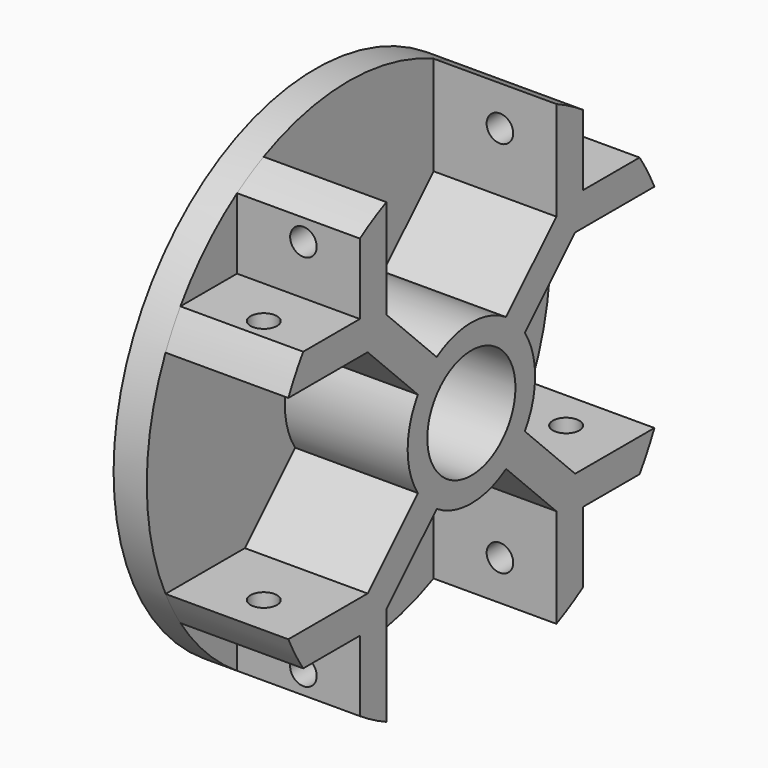
from build123d import *

# Parameters (mm, degrees)
F0_R            = 19
F1_DEPTH        = 2.5
F3_DEPTH        = 9.25
F4_R            = 1
F5_DEPTH        = 20
F5_COPIES_COUNT = 3
F5_COPIES_ANGLE = 180
F6_R            = 1
F7_DEPTH        = 20
F8_R            = 3
F9_DEPTH        = 2
F10_DEPTH       = 2
F11_R           = 4.15
F12_DEPTH       = 11.75


# Not quite as in the source:
# - a pattern or mirror of a feature is missing from the dataset's text; its kind, count and spacing are read off the source's solid


with BuildPart() as f1:
    # F0 (on Right) → F1 (new body)
    with BuildSketch(Plane.YZ):
        Circle(F0_R)
    extrude(amount=F1_DEPTH)

    # F2 (on face) → F3 (join)
    with BuildSketch(Plane.YZ.offset(2.5)):
        with BuildLine():
            ThreePointArc((-8, 17.2336879396), (-9.2763958902, 16.5815704711), (-10.5, 15.8350876221))
            Line((-10.5, 15.8350876221), (-10.5, 10.5))
            Line((-10.5, 10.5), (-15.8350876221, 10.5))
            ThreePointArc((-15.8350876221, 10.5), (-16.5815704711, 9.2763958902), (-17.2336879396, 8))
            Line((-17.2336879396, 8), (-9.767766953, 8))
            Line((-9.767766953, 8), (-5.0334316447, 3.2656646917))
            ThreePointArc((-5.0334316447, 3.2656646917), (-4.2426406871, 4.2426406871), (-3.2656646917, 5.0334316447))
            Line((-3.2656646917, 5.0334316447), (-8, 9.767766953))
            Line((-8, 9.767766953), (-8, 17.2336879396))
        make_face()
        with BuildLine():
            ThreePointArc((3.2656646917, 5.0334316447), (0, 6), (-3.2656646917, 5.0334316447))
            ThreePointArc((-3.2656646917, 5.0334316447), (-4.2426406871, 4.2426406871), (-5.0334316447, 3.2656646917))
            ThreePointArc((-5.0334316447, 3.2656646917), (-6, 0), (-5.0334316447, -3.2656646917))
            ThreePointArc((-5.0334316447, -3.2656646917), (-4.2426406871, -4.2426406871), (-3.2656646917, -5.0334316447))
            ThreePointArc((-3.2656646917, -5.0334316447), (0, -6), (3.2656646917, -5.0334316447))
            ThreePointArc((3.2656646917, -5.0334316447), (4.2426406871, -4.2426406871), (5.0334316447, -3.2656646917))
            ThreePointArc((5.0334316447, -3.2656646917), (5.7532855773, -1.7028520388), (6, 0))
            ThreePointArc((6, 0), (5.7532855773, 1.7028520388), (5.0334316447, 3.2656646917))
            ThreePointArc((5.0334316447, 3.2656646917), (4.2426406871, 4.2426406871), (3.2656646917, 5.0334316447))
        make_face()
        with BuildLine():
            ThreePointArc((10.5, 15.8350876221), (9.2763958902, 16.5815704711), (8, 17.2336879396))
            Line((8, 17.2336879396), (8, 9.767766953))
            Line((8, 9.767766953), (3.2656646917, 5.0334316447))
            ThreePointArc((3.2656646917, 5.0334316447), (4.2426406871, 4.2426406871), (5.0334316447, 3.2656646917))
            Line((5.0334316447, 3.2656646917), (9.767766953, 8))
            Line((9.767766953, 8), (17.2336879396, 8))
            ThreePointArc((17.2336879396, 8), (16.5815704711, 9.2763958902), (15.8350876221, 10.5))
            Line((15.8350876221, 10.5), (10.5, 10.5))
            Line((10.5, 10.5), (10.5, 15.8350876221))
        make_face()
        with BuildLine():
            ThreePointArc((15.8350876221, -10.5), (16.5815704711, -9.2763958902), (17.2336879396, -8))
            Line((17.2336879396, -8), (9.767766953, -8))
            Line((9.767766953, -8), (5.0334316447, -3.2656646917))
            ThreePointArc((5.0334316447, -3.2656646917), (4.2426406871, -4.2426406871), (3.2656646917, -5.0334316447))
            Line((3.2656646917, -5.0334316447), (8, -9.767766953))
            Line((8, -9.767766953), (8, -17.2336879396))
            ThreePointArc((8, -17.2336879396), (9.2763958902, -16.5815704711), (10.5, -15.8350876221))
            Line((10.5, -15.8350876221), (10.5, -10.5))
            Line((10.5, -10.5), (15.8350876221, -10.5))
        make_face()
        with BuildLine():
            Line((-9.767766953, -8), (-17.2336879396, -8))
            ThreePointArc((-17.2336879396, -8), (-16.5815704711, -9.2763958902), (-15.8350876221, -10.5))
            Line((-15.8350876221, -10.5), (-10.5, -10.5))
            Line((-10.5, -10.5), (-10.5, -15.8350876221))
            ThreePointArc((-10.5, -15.8350876221), (-9.2763958902, -16.5815704711), (-8, -17.2336879396))
            Line((-8, -17.2336879396), (-8, -9.767766953))
            Line((-8, -9.767766953), (-3.2656646917, -5.0334316447))
            ThreePointArc((-3.2656646917, -5.0334316447), (-4.2426406871, -4.2426406871), (-5.0334316447, -3.2656646917))
            Line((-5.0334316447, -3.2656646917), (-9.767766953, -8))
        make_face()
    extrude(amount=F3_DEPTH)

    # F4 (on face) → F5 (cut, symmetric)
    with BuildSketch(Plane(origin=(0, -8, 0), x_dir=(-1, 0, 0), z_dir=(0, 1, 0))):
        with Locations((-7.5, 14.2336879396)):
            Circle(F4_R)
    f5 = extrude(amount=F5_DEPTH, both=True, mode=Mode.SUBTRACT)

    # F5_copies: F5 ×3 about axis
    f5_copies_axis = Axis((0, 0, 0), (-1, 0, 0))
    for i in range(1, F5_COPIES_COUNT):
        add(f5.rotate(f5_copies_axis, i * F5_COPIES_ANGLE / (F5_COPIES_COUNT - 1)), mode=Mode.SUBTRACT)

    # F6 (on face) → F7 (cut, symmetric)
    with BuildSketch(Plane(origin=(0, 0, 8), x_dir=(1, 0, 0), z_dir=(0, 0, -1))):
        with Locations((7.5, 14.2336879396)):
            Circle(F6_R)
    extrude(amount=F7_DEPTH, both=True, mode=Mode.SUBTRACT)

    # F8 (on face) → F9 (join)
    with BuildSketch(Plane(origin=(0, 0, 0), x_dir=(0, -1, 0), z_dir=(-1, 0, 0))):
        with Locations((7.0710678119, 7.0710678119)):
            Circle(F8_R)
    extrude(amount=F9_DEPTH)

    # F8 (on face) → F10 (cut)
    with BuildSketch(Plane(origin=(0, 0, 0), x_dir=(0, -1, 0), z_dir=(-1, 0, 0))):
        with Locations((10, 0)):
            Circle(F8_R)
    extrude(amount=-F10_DEPTH, mode=Mode.SUBTRACT)

    # F11 (on face) → F12 (cut, through all)
    with BuildSketch(Plane.YZ.offset(11.75)):
        Circle(F11_R)
    extrude(amount=-F12_DEPTH, mode=Mode.SUBTRACT)


solid = f1.part
